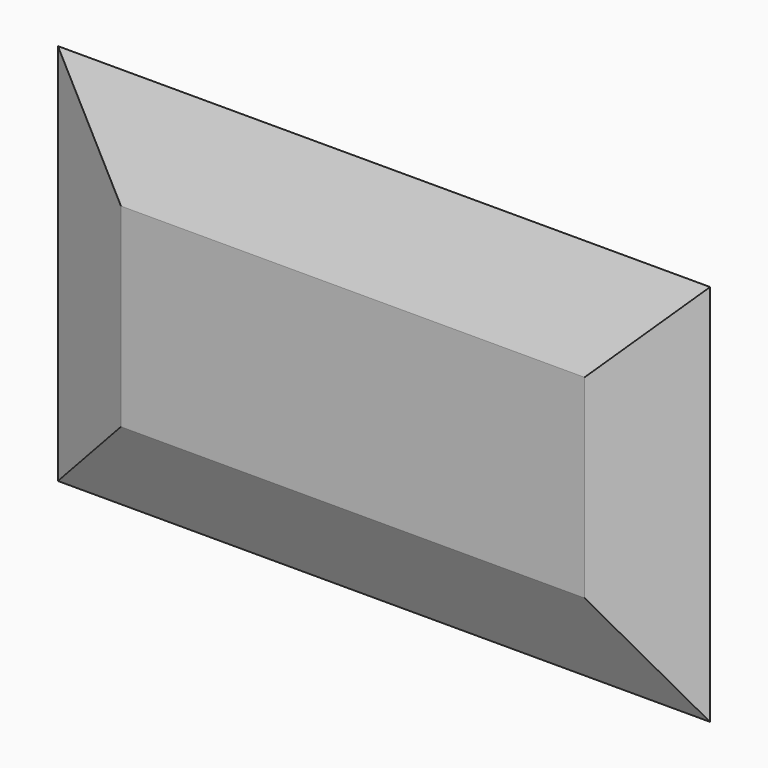
from build123d import *

# Parameters (mm, degrees)
F0_W        = 44.4469191134
F0_H        = 30.4321236908
F1_DEPTH    = 2.032
F2_T1_DEPTH = 70.5752182711
F2_T3_DEPTH = 56.5604228486
F3_T1_DEPTH = 60.6284503053
F3_T3_DEPTH = 46.6136548828


# Not quite as in the source:
# - a fillet or chamfer that OpenCascade refuses, or shapes differently, is made with other operations: its cross-section is extruded or revolved along the edge and cut away or added
# - a feature of the source that left no trace in its solid (it failed there, or was rolled back) is left out


with BuildPart() as f1:
    # F0 (on Front) → F1 (new body)
    with BuildSketch(Plane.XZ):
        with Locations((-32.5259137899, 4.3256785721)):
            Rectangle(F0_W, F0_H)
    extrude(amount=F1_DEPTH)

    # F2: chamfer of 5.08 on 4 edges, made by hand

    # F2_s2 → F2_t1 (cut)
    with BuildSketch(Plane.YZ.offset(-67.8135229254)):
        Polygon((3.048, 19.5417404175), (-2.032, 14.4617404175), (-2.032, 19.5417404175), align=None)
        Polygon((3.048, -10.8903832734), (-2.032, -5.8103832734), (-2.032, -10.8903832734), align=None)
    extrude(amount=F2_T1_DEPTH, mode=Mode.SUBTRACT)

    # F2_s4 → F2_t3 (cut)
    with BuildSketch(Plane.XY.offset(-23.9545328522)):
        Polygon((-54.7493733466, 3.048), (-49.6693733466, -2.032), (-54.7493733466, -2.032), align=None)
        Polygon((-10.3024542332, 3.048), (-15.3824542332, -2.032), (-10.3024542332, -2.032), align=None)
    extrude(amount=F2_T3_DEPTH, mode=Mode.SUBTRACT)

    # F3: chamfer of 5.08 on 4 edges, made by hand

    # F3_s2 → F3_t1 (cut)
    with BuildSketch(Plane.YZ.offset(-62.8401389426)):
        Polygon((1.5601024484, -9.4024857218), (-2.032, -0.7303832734), (-2.032, -5.8103832734), align=None)
        Polygon((1.5601024484, 18.0538428659), (-2.032, 9.3817404175), (-2.032, 14.4617404175), align=None)
    extrude(amount=F3_T1_DEPTH, mode=Mode.SUBTRACT)

    # F3_s4 → F3_t3 (cut)
    with BuildSketch(Plane.XY.offset(-18.9811488694)):
        Polygon((-53.261475795, 1.5601024484), (-44.5893733466, -2.032), (-49.6693733466, -2.032), align=None)
        Polygon((-11.7903517848, 1.5601024484), (-20.4624542332, -2.032), (-15.3824542332, -2.032), align=None)
    extrude(amount=F3_T3_DEPTH, mode=Mode.SUBTRACT)


solid = f1.part
